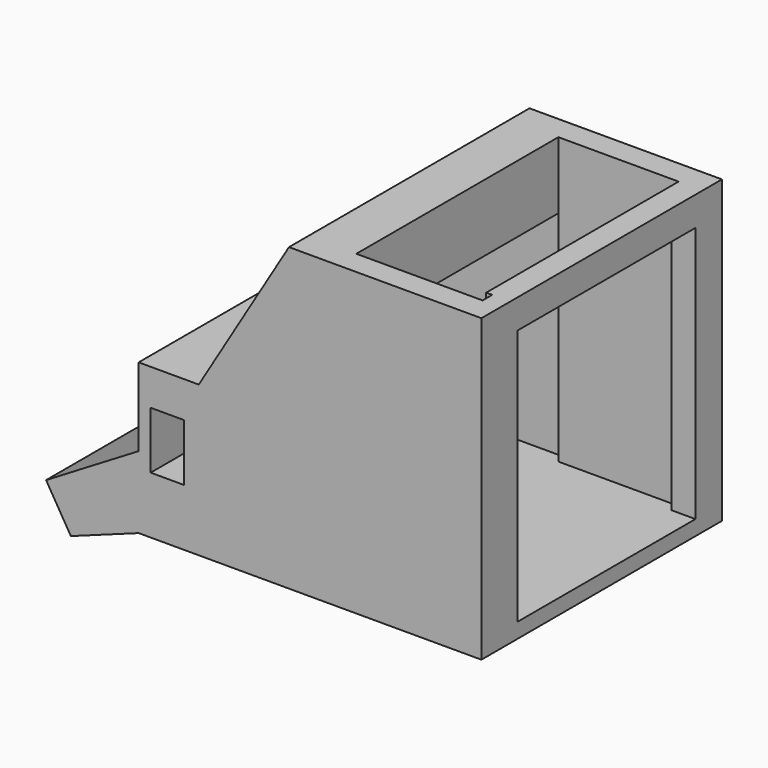
from build123d import *

# Parameters (mm, degrees)
F0_W      = 5.5
F0_H      = 9.5
F1_DEPTH  = 50
F2_T      = -2.5
F3_W      = 46
F3_H      = 4
F4_DEPTH  = 18
F5_DEPTH  = 30
F6_W      = 2
F6_H      = 3
F7_DEPTH  = 42.640873421
F8_W      = 20
F8_H      = 42
F9_DEPTH  = 4.859126579
F10_W     = 1.7037652433
F10_H     = 3.2813884318
F11_DEPTH = 45
F12_W     = 1
F12_H     = 2
F13_DEPTH = 5
F14_DEPTH = 42.640873421
F15_DEPTH = 5
F16_DEPTH = 3
F17_DEPTH = 2
F20_DEPTH = 50
F21_DEPTH = 25
F22_DEPTH = 15
F23_DEPTH = 0.5
F24_DEPTH = 3
F25_DEPTH = 2
F26_R     = 2
F27_DEPTH = 6


with BuildPart() as f1:
    # F0 (on Front) → F1 (new body)
    with BuildSketch(Plane.XZ):
        Polygon((0, 12), (0, 0), (20, 0), (20, 25), (10, 25), (0, 25), align=None)
        with Locations((4.75, 14.25)):
            Rectangle(F0_W, F0_H, mode=Mode.SUBTRACT)
        Polygon((20, 25), (20, 0), (25, 0), (25, 50), (10, 25), align=None)
        Polygon((-11.2763114494, -4.1042417199), (0, 0), (0, 12), (-15.3952030634, 2.7539454948), align=None)
    extrude(amount=F1_DEPTH)

    # F2
    f2_openings = [f1.faces().sort_by_distance(p)[0] for p in [
        (25, -25, 25),
    ]]
    offset(amount=F2_T, openings=f2_openings, kind=Kind.INTERSECTION)

    # F3 (on face) → F4 (cut)
    with BuildSketch(Plane(origin=(-10.0986787248, 0, -6.0650667312), x_dir=(0, -1, 0), z_dir=(-0.8572734018, 0, -0.5148614518))):
        with Locations((25, 6.2872808221)):
            Rectangle(F3_W, F3_H)
    extrude(amount=-F4_DEPTH, mode=Mode.SUBTRACT)

    # F5 (add): a face of the model
    f5_faces = [f1.faces().sort_by_distance(p)[0] for p in [
        (25, -25, 0.7071067812),
    ]]
    extrude(f5_faces, amount=F5_DEPTH)

    # F6 (on face) → F7 (join, through all)
    with BuildSketch(Plane(origin=(0, 0, 45.140873421), x_dir=(1, 0, 0), z_dir=(0, 0, -1))):
        with Locations((54, 46)):
            Rectangle(F6_W, F6_H)
        with Locations((54, 4)):
            Rectangle(F6_W, F6_H)
    extrude(amount=F7_DEPTH)

    # F8 (on face) → F9 (cut, through all)
    with BuildSketch(Plane.XY.offset(50)):
        with Locations((43, -25)):
            Rectangle(F8_W, F8_H)
    extrude(amount=-F9_DEPTH, mode=Mode.SUBTRACT)

    # F10 (on face) → F11 (join, through all)
    with BuildSketch(Plane.XZ.offset(2.5)):
        with Locations((32.1481173784, 43.5001792051)):
            Rectangle(F10_W, F10_H)
    extrude(amount=F11_DEPTH)

    # F12 (on face) → F13 (cut)
    with BuildSketch(Plane.XY.offset(50)):
        with Locations((53.5, -45)):
            Rectangle(F12_W, F12_H)
    extrude(amount=-F13_DEPTH, mode=Mode.SUBTRACT)

    # F14 (add, through all): faces of the model
    f14_faces = [f1.faces().sort_by_distance(p)[0] for p in [
        (43, -46.75, 45.140873421),
        (43, -3.25, 45.140873421),
    ]]
    extrude(f14_faces, amount=F14_DEPTH)

    # F15 (add): a face of the model
    f15_faces = [f1.faces().sort_by_distance(p)[0] for p in [
        (55, -25, 0.7071067812),
    ]]
    extrude(f15_faces, amount=F15_DEPTH)

    # F16 (add): a face of the model
    f16_faces = [f1.faces().sort_by_distance(p)[0] for p in [
        (32.1481173784, -25, 41.8594849892),
    ]]
    extrude(f16_faces, amount=F16_DEPTH)

    # F17 (add): a face of the model
    f17_faces = [f1.faces().sort_by_distance(p)[0] for p in [
        (56.5014165477, -44.5, 23.810402831),
    ]]
    extrude(f17_faces, amount=F17_DEPTH)

    # F19 (on face) → F20 (join)
    with BuildSketch(Plane.XZ.offset(50)):
        Polygon((-11.2763114494, -4.1042417199), (-15.3952030634, 2.7539454948), (-19.6083863192, -2.1957097309), (-23.1083863192, -3.9201829974), (-21.6654660693, -6.8880073104), align=None)
    extrude(amount=-F20_DEPTH)

    # F18 (on face) → F21 (cut)
    with BuildSketch(Plane(origin=(-5.2965243386, 0, 8.819012226), x_dir=(0.8572734018, 0, 0.5148614518), z_dir=(-0.5148614518, 0, 0.8572734018))):
        Polygon((-33.7799977267, -50), (-11.7799977267, -50), (-33.7799977267, -28), align=None)
        Polygon((-33.7799977267, -22), (-11.7799977267, 0), (-33.7799977267, 0), align=None)
    extrude(amount=-F21_DEPTH, mode=Mode.SUBTRACT)

    # F22 (cut): a face of the model
    f22_faces = [f1.faces().sort_by_distance(p)[0] for p in [
        (-22.3892898276, -25, -5.3992335904),
    ]]
    extrude(f22_faces, amount=-F22_DEPTH, mode=Mode.SUBTRACT)

    # F23 (add): a face of the model
    f23_faces = [f1.faces().sort_by_distance(p)[0] for p in [
        (-21.2912627093, -25, -3.0248741153),
    ]]
    extrude(f23_faces, amount=-F23_DEPTH)

    # F24 (cut): a face of the model
    f24_faces = [f1.faces().sort_by_distance(p)[0] for p in [
        (60, -25, 0.7071067812),
    ]]
    extrude(f24_faces, amount=-F24_DEPTH, mode=Mode.SUBTRACT)

    # F25 (add): a face of the model
    f25_faces = [f1.faces().sort_by_distance(p)[0] for p in [
        (6.25, -25, 21.5),
    ]]
    extrude(f25_faces, amount=F25_DEPTH)

    # F26 (on face) → F27 (cut)
    with BuildSketch(Plane.XY.offset(25)):
        with Locations((5, -25)):
            Circle(F26_R)
    extrude(amount=-F27_DEPTH, mode=Mode.SUBTRACT)


solid = f1.part
